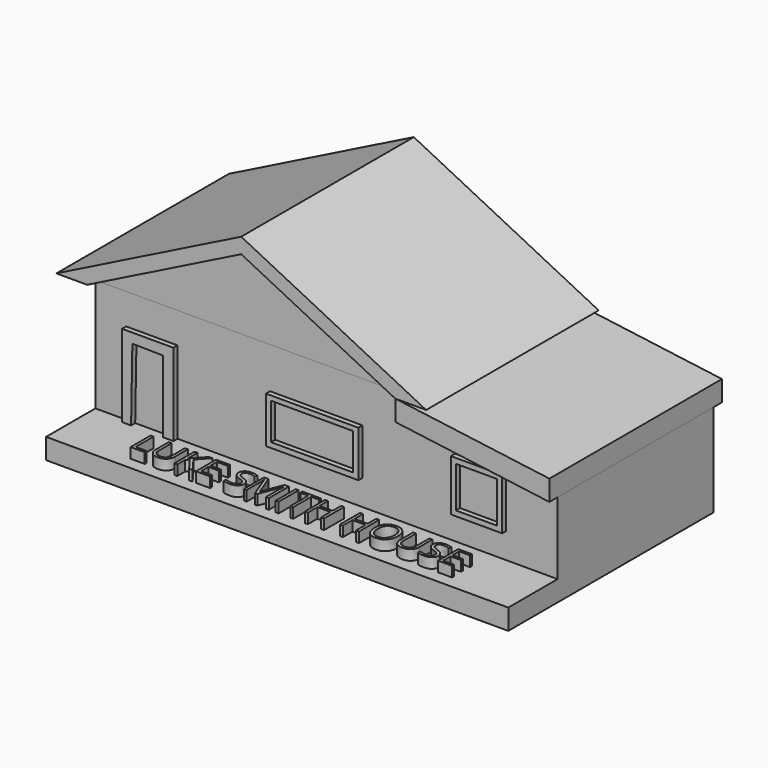
from build123d import *

# Parameters (mm, degrees)
F1_DEPTH      = 6096
F1_DEPTH_BACK = 304.8
F2_DEPTH      = 5791.2
F3_DEPTH      = 6096
F3_DEPTH_BACK = 304.8
F0_W          = 2743.2
F0_H          = 1371.6
F0_W_2        = 1524
F0_H_2        = 1524
F4_DEPTH      = 5791.2
F5_DEPTH      = 5943.6
F6_DEPTH      = 5791.2
F0_W_3        = 2438.4
F0_H_3        = 1081.8144973755
F0_W_4        = 1219.2
F0_H_4        = 1219.2
F7_DEPTH      = 5943.6
F8_DEPTH      = 5791.2
F0_W_5        = 4572
F0_H_5        = 609.6
F9_DEPTH      = 7620
F10_TEXT_SIZE = 1042.7369011773
F11_DEPTH     = 304.8


# Not quite as in the source:
# - Text() gives the source's letters only with a copy of the font that has no kerning and outlines rounded to 1/6400 em; it was checked with that copy


with BuildPart() as f1:
    # F0 (on Front) → F1 (new body, two sides)
    with BuildSketch(Plane.XZ) as f1_sk:
        Polygon((-5486.4, 0), (-4572, 0), (0, 2286), (4572, 0), (5486.4, 0), (0, 2743.2), align=None)
    extrude(amount=F1_DEPTH)
    extrude(f1_sk.sketch, amount=-F1_DEPTH_BACK)

    # F0 (on Front) → F2 (join)
    with BuildSketch(Plane.XZ):
        Polygon((-4572, 0), (0, 0), (4572, 0), (0, 2286), align=None)
    extrude(amount=F2_DEPTH)


with BuildPart() as f3:
    # F0 (on Front) → F3 (new body, two sides)
    with BuildSketch(Plane.XZ) as f3_sk:
        Polygon((9144, -603.2345459073), (4572, 0), (4572, -609.6), (9144, -1212.8345459073), align=None)
    extrude(amount=F3_DEPTH)
    extrude(f3_sk.sketch, amount=-F3_DEPTH_BACK)


with BuildPart() as f4:
    # F0 (on Front) → F4 (new body)
    with BuildSketch(Plane.XZ):
        Polygon((4572, 0), (0, 0), (-4572, 0), (-4572, -3352.8), (-3657.6, -3352.8), (-3657.6, -914.4), (-2133.6041321198, -914.4), (-2133.6041321198, -3352.8), (4572, -3352.8), (4572, -609.6), align=None)
        with Locations((1981.2, -1905)):
            Rectangle(F0_W, F0_H, mode=Mode.SUBTRACT)
        Polygon((9144, -1212.8345459073), (4572, -609.6), (4572, -3352.8), (9144, -3352.8), align=None)
        with Locations((6858, -1828.8)):
            Rectangle(F0_W_2, F0_H_2, mode=Mode.SUBTRACT)
    extrude(amount=F4_DEPTH)

    # F0 (on Front) → F5 (join)
    with BuildSketch(Plane.XZ):
        Polygon((-3657.6, -914.4), (-3657.6, -3352.8), (-3390.185547414, -3352.8), (-3352.6648645708, -1203.2415195537), (-2438.4041321198, -1219.2), (-2438.4041321198, -3352.8), (-2133.6041321198, -3352.8), (-2133.6041321198, -914.4), align=None)
    extrude(amount=F5_DEPTH)

    # F0 (on Front) → F6 (join)
    with BuildSketch(Plane.XZ):
        Polygon((-3352.6648645708, -1203.2415195537), (-3390.185547414, -3352.8), (-2438.4041321198, -3352.8), (-2438.4041321198, -1219.2), align=None)
    extrude(amount=F6_DEPTH)

    # F0 (on Front) → F7 (join)
    with BuildSketch(Plane.XZ):
        with Locations((1981.2, -1905)):
            Rectangle(F0_W, F0_H)
        with Locations((1981.2, -1897.4927513123)):
            Rectangle(F0_W_3, F0_H_3, mode=Mode.SUBTRACT)
        with Locations((6858, -1828.8)):
            Rectangle(F0_W_2, F0_H_2)
        with Locations((6858, -1828.8)):
            Rectangle(F0_W_4, F0_H_4, mode=Mode.SUBTRACT)
    extrude(amount=F7_DEPTH)

    # F0 (on Front) → F8 (join)
    with BuildSketch(Plane.XZ):
        with Locations((1981.2, -1897.4927513123)):
            Rectangle(F0_W_3, F0_H_3)
        with Locations((6858, -1828.8)):
            Rectangle(F0_W_4, F0_H_4)
    extrude(amount=F8_DEPTH)

    # F0 (on Front) → F9 (join)
    with BuildSketch(Plane.XZ):
        Polygon((-3657.6, -3352.8), (-4572, -3352.8), (-4572, -3962.4), (4572, -3962.4), (4572, -3352.8), (-2133.6041321198, -3352.8), (-2438.4041321198, -3352.8), (-3390.185547414, -3352.8), align=None)
        with Locations((6858, -3657.6)):
            Rectangle(F0_W_5, F0_H_5)
    extrude(amount=F9_DEPTH)

    # F10 (on face) → F11 (join)
    with BuildSketch(Plane.XY.offset(-3352.8)):
        with Locations((-2456.8483829498, -7255.0420761108)):
            Text('LUKE SMITH HOUSE', F10_TEXT_SIZE, font='Open Sans', text_align=(TextAlign.LEFT, TextAlign.BOTTOM))
    extrude(amount=F11_DEPTH)


solid = Compound([f1.part, f3.part, f4.part])
